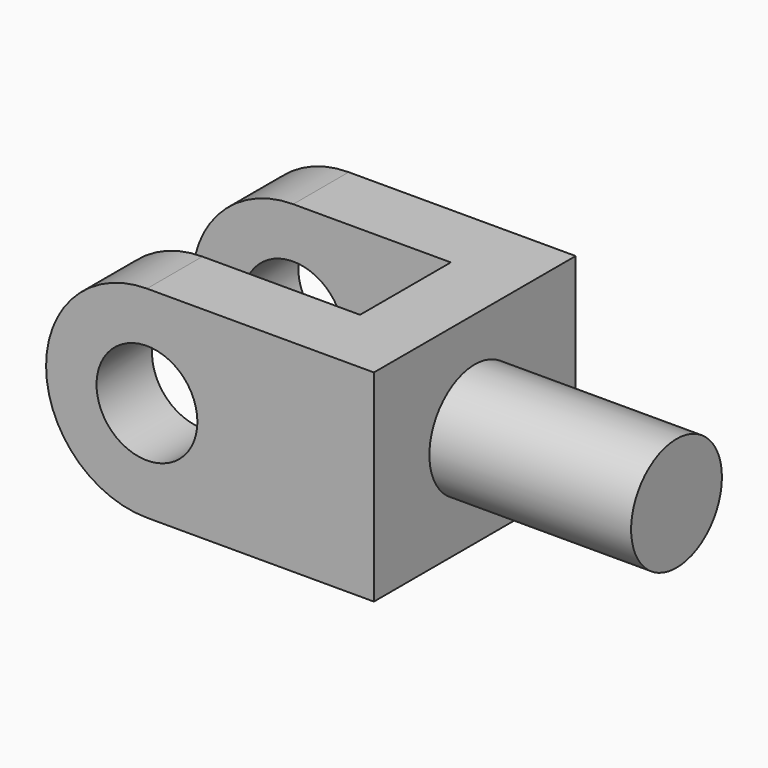
from build123d import *

# Parameters (mm, degrees)
F1_DEPTH = 812.8
F2_R     = 203.2
F3_DEPTH = 1016.001
F4_R     = 228.6
F5_DEPTH = 812.8


# Not quite as in the source:
# - a feature names something its author has since deleted; it is built from what else it names


with BuildPart() as f1:
    # F0 (on Top) → F1 (new body)
    with BuildSketch(Plane.XY):
        Polygon((0, -279.4), (0, 0), (0, 736.6), (-1320.8, 736.6), (-1320.8, 457.2), (-279.4, 457.2), (-279.4, 0), (-1320.8, 0), (-1320.8, -279.4), align=None)
    extrude(amount=F1_DEPTH)

    # F2 (on face) → F3 (cut, through all)
    with BuildSketch(Plane.XZ.offset(279.4)):
        with BuildLine():
            ThreePointArc((-1320.8, 406.4), (-1201.7681958742, 693.7681958742), (-914.4, 812.8))
            Line((-914.4, 812.8), (-1320.8, 812.8))
            Line((-1320.8, 812.8), (-1320.8, 406.4))
        make_face()
        with BuildLine():
            ThreePointArc((-914.4, 0), (-1201.7681958742, 119.0318041258), (-1320.8, 406.4))
            Line((-1320.8, 406.4), (-1320.8, 0))
            Line((-1320.8, 0), (-914.4, 0))
        make_face()
        with Locations((-914.4, 406.4)):
            Circle(F2_R)
    extrude(amount=-F3_DEPTH, mode=Mode.SUBTRACT)

    # F4 (on face) → F5 (join)
    with BuildSketch(Plane.YZ):
        with Locations((228.6, 406.4)):
            Circle(F4_R)
    extrude(amount=F5_DEPTH)


solid = f1.part
